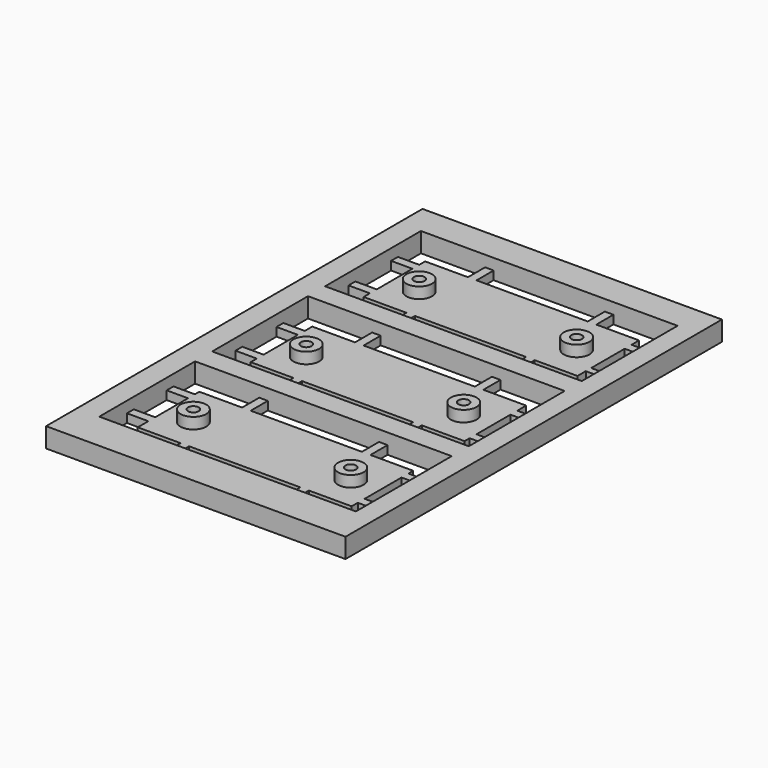
from build123d import *

# Parameters (mm, degrees)
F0_R     = 3
F0_W     = 2
F0_H     = 5
F0_W_2   = 5
F0_H_2   = 2
F0_H_3   = 2.0107477903
F0_H_4   = 1.5826318413
F1_DEPTH = 2
F0_H_5   = 1.9926615059
F2_W     = 70
F2_H     = 110
F2_W_2   = 60
F2_H_2   = 28
F3_DEPTH = 4.6
F0_R_2   = 1.25
F4_DEPTH = 4.6


with BuildPart() as f1:
    # F0 (on Top) → F1 (new body)
    with BuildSketch(Plane.XY):
        Polygon((-4.260212779, 31.3345443402), (-14.260212779, 31.3345443402), (-14.260212779, 29.606844902), (-14.260212779, 27.606844902), (-14.260212779, 22.3345443402), (-14.260212779, 20.3345443402), (-14.260212779, 17.1737267151), (-14.260212779, 15.1737267151), (-14.260212779, 13.3345443402), (-4.260212779, 13.3345443402), (-2.260212779, 13.3345443402), (8.7358048186, 13.3345443402), (10.7358048186, 13.3345443402), (23.739787221, 13.3345443402), (25.739787221, 13.3345443402), (35.739787221, 13.3345443402), (35.739787221, 15.7596264035), (35.739787221, 17.3422582448), (35.739787221, 20.3345443402), (35.739787221, 22.3345443402), (35.739787221, 27.1184686571), (35.739787221, 29.1292164475), (35.739787221, 31.3345443402), (25.739787221, 31.3345443402), (23.739787221, 31.3345443402), (10.739787221, 31.3345443402), (8.739787221, 31.3345443402), (-2.260212779, 31.3345443402), align=None)
        with Locations((-7.660212779, 21.3345443402)):
            Circle(F0_R, mode=Mode.SUBTRACT)
        with Locations((29.139787221, 21.3345443402)):
            Circle(F0_R, mode=Mode.SUBTRACT)
        with Locations((-3.260212779, 33.8345443402)):
            Rectangle(F0_W, F0_H)
        with Locations((-16.760212779, 28.606844902)):
            Rectangle(F0_W_2, F0_H_2)
        with Locations((24.739787221, 33.8345443402)):
            Rectangle(F0_W, F0_H)
        with Locations((-16.760212779, 16.1737267151)):
            Rectangle(F0_W_2, F0_H_2)
        with Locations((38.239787221, 28.1238425523)):
            Rectangle(F0_W_2, F0_H_3)
        with Locations((-3.260212779, 10.8345443402)):
            Rectangle(F0_W, F0_H)
        with Locations((38.239787221, 16.5509423241)):
            Rectangle(F0_W_2, F0_H_4)
        with Locations((24.739787221, 10.8345443402)):
            Rectangle(F0_W, F0_H)
    extrude(amount=F1_DEPTH)

    # F0 (on Top) → F4 (join)
    with BuildSketch(Plane.XY):
        with Locations((-7.660212779, 21.3345443402)):
            Circle(F0_R)
        with Locations((-7.660212779, 21.3345443402)):
            Circle(F0_R_2, mode=Mode.SUBTRACT)
        with Locations((29.139787221, 21.3345443402)):
            Circle(F0_R)
        with Locations((29.139787221, 21.3345443402)):
            Circle(F0_R_2, mode=Mode.SUBTRACT)
    extrude(amount=F4_DEPTH)


with BuildPart() as f1b:
    # F0 (on Top) → F1, piece 2 (new body)
    with BuildSketch(Plane.XY):
        Polygon((-4.260212779, -1.6654556598), (-14.260212779, -1.6654556598), (-14.260212779, -3.8577791788), (-14.260212779, -5.8577791788), (-14.260212779, -10.6654556598), (-14.260212779, -12.6654556598), (-14.260212779, -15.8761590719), (-14.260212779, -17.8688205779), (-14.260212779, -19.6654556598), (-4.260212779, -19.6654556598), (-2.260212779, -19.6654556598), (8.7807420641, -19.6654556598), (10.7807420641, -19.6654556598), (23.739787221, -19.6654556598), (25.739787221, -19.6654556598), (35.739787221, -19.6654556598), (35.739787221, -18.1903596967), (35.739787221, -16.1903596967), (35.739787221, -12.6654556598), (35.739787221, -10.6654556598), (35.739787221, -6.2599289231), (35.739787221, -4.2599289231), (35.739787221, -1.6654556598), (25.739787221, -1.6654556598), (23.739787221, -1.6654556598), (10.739787221, -1.6654556598), (8.739787221, -1.6654556598), (-2.260212779, -1.6654556598), align=None)
        with Locations((-7.660212779, -11.6654556598)):
            Circle(F0_R, mode=Mode.SUBTRACT)
        with Locations((29.139787221, -11.6654556598)):
            Circle(F0_R, mode=Mode.SUBTRACT)
        with Locations((-3.260212779, 0.8345443402)):
            Rectangle(F0_W, F0_H)
        with Locations((-16.760212779, -4.8577791788)):
            Rectangle(F0_W_2, F0_H_2)
        with Locations((24.739787221, 0.8345443402)):
            Rectangle(F0_W, F0_H)
        with Locations((-16.760212779, -16.8724898249)):
            Rectangle(F0_W_2, F0_H_5)
        with Locations((38.239787221, -5.2599289231)):
            Rectangle(F0_W_2, F0_H_2)
        with Locations((-3.260212779, -22.1654556598)):
            Rectangle(F0_W, F0_H)
        with Locations((38.239787221, -17.1903596967)):
            Rectangle(F0_W_2, F0_H_2)
        with Locations((24.739787221, -22.1654556598)):
            Rectangle(F0_W, F0_H)
    extrude(amount=F1_DEPTH)


with BuildPart() as f1c:
    # F0 (on Top) → F1, piece 3 (new body)
    with BuildSketch(Plane.XY):
        Polygon((-4.260212779, -34.6654556598), (-14.260212779, -34.6654556598), (-14.260212779, -35.9602573812), (-14.260212779, -37.9602573812), (-14.260212779, -41.6654556598), (-14.260212779, -43.6654556598), (-14.260212779, -47.5723225176), (-14.260212779, -49.5723225176), (-14.260212779, -52.6654556598), (-4.260212779, -52.6654556598), (-2.260212779, -52.6654556598), (8.3012469113, -52.6654556598), (10.3012469113, -52.6654556598), (23.739787221, -52.6654556598), (25.739787221, -52.6654556598), (35.739787221, -52.6654556598), (35.739787221, -50.8625470102), (35.739787221, -48.8625470102), (35.739787221, -45.6654556598), (35.739787221, -43.6654556598), (35.739787221, -38.0775518715), (35.739787221, -36.0775518715), (35.739787221, -34.6654556598), (25.739787221, -34.6654556598), (23.739787221, -34.6654556598), (10.7358048186, -34.6654556598), (8.7358048186, -34.6654556598), (-2.260212779, -34.6654556598), align=None)
        with Locations((-7.660212779, -44.6654556598)):
            Circle(F0_R, mode=Mode.SUBTRACT)
        with Locations((29.139787221, -44.6654556598)):
            Circle(F0_R, mode=Mode.SUBTRACT)
        with Locations((-3.260212779, -32.1654556598)):
            Rectangle(F0_W, F0_H)
        with Locations((-16.760212779, -36.9602573812)):
            Rectangle(F0_W_2, F0_H_2)
        with Locations((24.739787221, -32.1654556598)):
            Rectangle(F0_W, F0_H)
        with Locations((-16.760212779, -48.5723225176)):
            Rectangle(F0_W_2, F0_H_2)
        with Locations((38.239787221, -37.0775518715)):
            Rectangle(F0_W_2, F0_H_2)
        with Locations((-3.260212779, -55.1654556598)):
            Rectangle(F0_W, F0_H)
        with Locations((38.239787221, -49.8625470102)):
            Rectangle(F0_W_2, F0_H_2)
        with Locations((24.739787221, -55.1654556598)):
            Rectangle(F0_W, F0_H)
    extrude(amount=F1_DEPTH)


with BuildPart() as f3:
    # F2 (on Top) → F3 (new body)
    with BuildSketch(Plane.XY):
        with Locations((10.5093383789, -11.6654556598)):
            Rectangle(F2_W, F2_H)
        with Locations((10.739787221, -43.6654556598)):
            Rectangle(F2_W_2, F2_H_2, mode=Mode.SUBTRACT)
        with Locations((10.739787221, -10.6654556598)):
            Rectangle(F2_W_2, F2_H_2, mode=Mode.SUBTRACT)
        with Locations((10.739787221, 22.3345443402)):
            Rectangle(F2_W_2, F2_H_2, mode=Mode.SUBTRACT)
    extrude(amount=F3_DEPTH)


with BuildPart() as f4:
    # F0 (on Top) → F4, piece 2 (new body)
    with BuildSketch(Plane.XY):
        with Locations((-7.660212779, -11.6654556598)):
            Circle(F0_R)
        with Locations((-7.660212779, -11.6654556598)):
            Circle(F0_R_2, mode=Mode.SUBTRACT)
    extrude(amount=F4_DEPTH)


with BuildPart() as f4b:
    # F0 (on Top) → F4, piece 3 (new body)
    with BuildSketch(Plane.XY):
        with Locations((29.139787221, -11.6654556598)):
            Circle(F0_R)
        with Locations((29.139787221, -11.6654556598)):
            Circle(F0_R_2, mode=Mode.SUBTRACT)
    extrude(amount=F4_DEPTH)


with BuildPart() as f4c:
    # F0 (on Top) → F4, piece 4 (new body)
    with BuildSketch(Plane.XY):
        with Locations((-7.660212779, -44.6654556598)):
            Circle(F0_R)
        with Locations((-7.660212779, -44.6654556598)):
            Circle(F0_R_2, mode=Mode.SUBTRACT)
    extrude(amount=F4_DEPTH)


with BuildPart() as f4d:
    # F0 (on Top) → F4, piece 5 (new body)
    with BuildSketch(Plane.XY):
        with Locations((29.139787221, -44.6654556598)):
            Circle(F0_R)
        with Locations((29.139787221, -44.6654556598)):
            Circle(F0_R_2, mode=Mode.SUBTRACT)
    extrude(amount=F4_DEPTH)


solid = Compound([f1.part, f1b.part, f1c.part, f3.part, f4.part, f4b.part, f4c.part, f4d.part])
